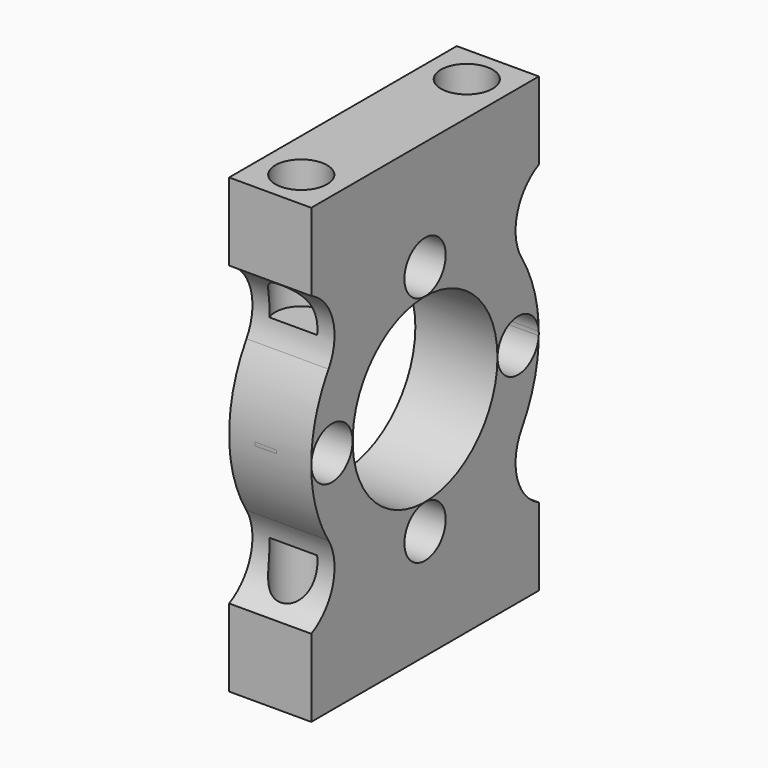
from build123d import *

# Parameters (mm, degrees)
F0_R        = 1
F0_R_2      = 7
F1_DEPTH    = 6.35
F2_T1_DEPTH = 6.35
F3_R        = 1.995
F4_DEPTH    = 4.35
F5_R        = 2
F6_DEPTH    = 10
F7_R        = 2
F8_DEPTH    = 10


# Not quite as in the source:
# - a fillet or chamfer that OpenCascade refuses, or shapes differently, is made with other operations: its cross-section is extruded or revolved along the edge and cut away or added


with BuildPart() as f1:
    # F0 (on Right) → F1 (new body)
    with BuildSketch(Plane.YZ):
        with BuildLine():
            ThreePointArc((-11, 11.5), (-8.5663313628, 10.4710489148), (-6.4168428396, 8.9344349554))
            ThreePointArc((-6.4168428396, 8.9344349554), (-11, 0), (-6.4168428396, -8.9344349554))
            ThreePointArc((-6.4168428396, -8.9344349554), (-8.5663313628, -10.4710489148), (-11, -11.5))
            Line((-11, -11.5), (-11, -17.5))
            Line((-11, -17.5), (11, -17.5))
            Line((11, -17.5), (11, -11.5))
            ThreePointArc((11, -11.5), (8.5663313628, -10.4710489148), (6.4168428396, -8.9344349554))
            ThreePointArc((6.4168428396, -8.9344349554), (11, 0), (6.4168428396, 8.9344349554))
            ThreePointArc((6.4168428396, 8.9344349554), (8.5663313628, 10.4710489148), (11, 11.5))
            Line((11, 11.5), (11, 17.5))
            Line((11, 17.5), (-11, 17.5))
            Line((-11, 17.5), (-11, 11.5))
        make_face()
        with Locations((0, -9)):
            Circle(F0_R, mode=Mode.SUBTRACT)
        with Locations((-9, 0)):
            Circle(F0_R, mode=Mode.SUBTRACT)
        Circle(F0_R_2, mode=Mode.SUBTRACT)
        with Locations((9, 0)):
            Circle(F0_R, mode=Mode.SUBTRACT)
        with Locations((0, 9)):
            Circle(F0_R, mode=Mode.SUBTRACT)
    extrude(amount=F1_DEPTH)

    # F2: fillet of radius 4 on 4 edges, made by hand

    # F2_s2 → F2_t1 (join)
    with BuildSketch(Plane.YZ):
        with BuildLine():
            ThreePointArc((-10.9998249992, 11.500359687), (-8.9067871665, 9.0142668997), (-9.3494629478, 5.7947167962))
            Line((-9.3494629478, 5.7947167962), (-9.0093791138, 5.5839357582))
            ThreePointArc((-9.0093791138, 5.5839357582), (-7.7456923262, 7.2361578693), (-6.1834406461, 8.6094594545))
            Line((-6.1834406461, 8.6094594545), (-6.1497385524, 9.2323291646))
            ThreePointArc((-6.1497385524, 9.2323291646), (-8.3709064916, 10.8201832442), (-10.8247773704, 11.8601429381))
            Line((-10.8247773704, 11.8601429381), (-10.9998249992, 11.500359687))
        make_face()
        with BuildLine():
            ThreePointArc((-9.3494629478, -5.7947167962), (-8.9067871665, -9.0142668997), (-10.9998249992, -11.500359687))
            Line((-10.9998249992, -11.500359687), (-10.8247773704, -11.8601429381))
            ThreePointArc((-10.8247773704, -11.8601429381), (-8.3709064916, -10.8201832442), (-6.1497385524, -9.2323291646))
            Line((-6.1497385524, -9.2323291646), (-6.1834406461, -8.6094594545))
            ThreePointArc((-6.1834406461, -8.6094594545), (-7.7456923262, -7.2361578693), (-9.0093791138, -5.5839357582))
            Line((-9.0093791138, -5.5839357582), (-9.3494629478, -5.7947167962))
        make_face()
        with BuildLine():
            ThreePointArc((10.9998249992, -11.500359687), (8.9067871665, -9.0142668997), (9.3494629478, -5.7947167962))
            Line((9.3494629478, -5.7947167962), (9.0093791138, -5.5839357582))
            ThreePointArc((9.0093791138, -5.5839357582), (7.7456923262, -7.2361578693), (6.1834406461, -8.6094594545))
            Line((6.1834406461, -8.6094594545), (6.1497385524, -9.2323291646))
            ThreePointArc((6.1497385524, -9.2323291646), (8.3709064916, -10.8201832442), (10.8247773704, -11.8601429381))
            Line((10.8247773704, -11.8601429381), (10.9998249992, -11.500359687))
        make_face()
        with BuildLine():
            ThreePointArc((10.9998249992, 11.500359687), (8.9067871665, 9.0142668997), (9.3494629478, 5.7947167962))
            Line((9.3494629478, 5.7947167962), (9.0093791138, 5.5839357582))
            ThreePointArc((9.0093791138, 5.5839357582), (7.7456923262, 7.2361578693), (6.1834406461, 8.6094594545))
            Line((6.1834406461, 8.6094594545), (6.1497385524, 9.2323291646))
            ThreePointArc((6.1497385524, 9.2323291646), (8.3709064916, 10.8201832442), (10.8247773704, 11.8601429381))
            Line((10.8247773704, 11.8601429381), (10.9998249992, 11.500359687))
        make_face()
    extrude(amount=F2_T1_DEPTH)

    # F3 (on face) → F4 (cut)
    with BuildSketch(Plane.YZ.offset(6.35)):
        with Locations((0, 9)):
            Circle(F3_R)
        with Locations((9, 0)):
            Circle(F3_R)
        with Locations((0, -9)):
            Circle(F3_R)
        with Locations((-9, 0)):
            Circle(F3_R)
    extrude(amount=-F4_DEPTH, mode=Mode.SUBTRACT)

    # F5 (on face) → F6 (cut)
    with BuildSketch(Plane.XY.offset(17.5)):
        with Locations((3.175, 8)):
            Circle(F5_R)
        with Locations((3.175, -8)):
            Circle(F5_R)
    extrude(amount=-F6_DEPTH, mode=Mode.SUBTRACT)

    # F7 (on face) → F8 (cut)
    with BuildSketch(Plane(origin=(0, 0, -17.5), x_dir=(1, 0, 0), z_dir=(0, 0, -1))):
        with Locations((3.175, 8)):
            Circle(F7_R)
        with Locations((3.175, -8)):
            Circle(F7_R)
    extrude(amount=-F8_DEPTH, mode=Mode.SUBTRACT)


solid = f1.part
